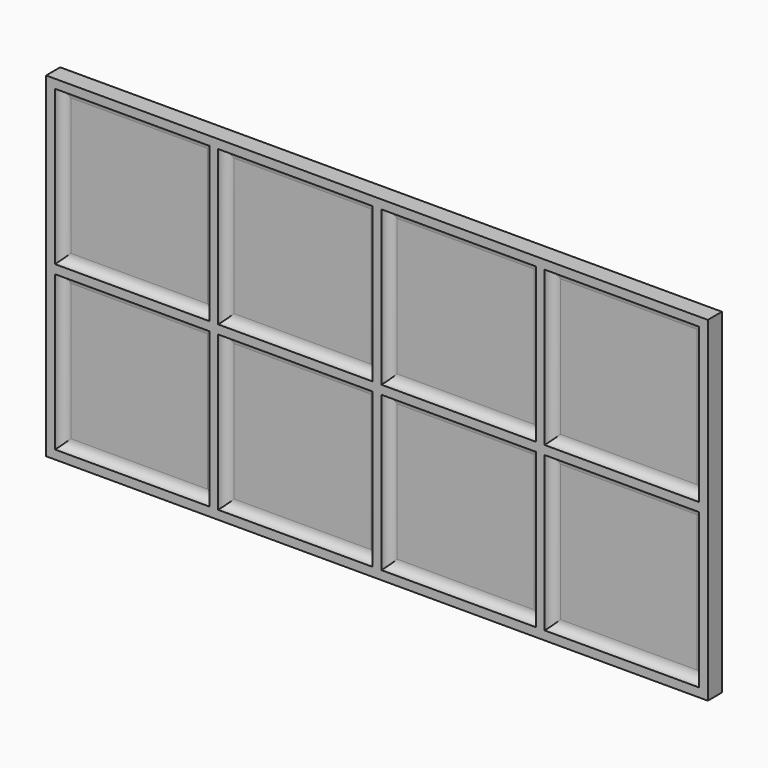
from build123d import *

# Parameters (mm, degrees)
F0_W     = 150
F0_H     = 76
F0_W_2   = 35
F0_H_2   = 35
F1_DEPTH = 2
F2_DEPTH = 4
F3_R     = 1.99999


# Not quite as in the source:
# - a fillet or chamfer is up to 0.001 mm smaller than in the source, because OpenCascade refuses the exact size


with BuildPart() as f1:
    # F0 (on Front) → F1 (new body)
    with BuildSketch(Plane.XZ):
        Rectangle(F0_W, F0_H)
        with Locations((-55.5, -18.5)):
            Rectangle(F0_W_2, F0_H_2, mode=Mode.SUBTRACT)
        with Locations((-18.5, -18.5)):
            Rectangle(F0_W_2, F0_H_2, mode=Mode.SUBTRACT)
        with Locations((18.5, -18.5)):
            Rectangle(F0_W_2, F0_H_2, mode=Mode.SUBTRACT)
        with Locations((55.5, -18.5)):
            Rectangle(F0_W_2, F0_H_2, mode=Mode.SUBTRACT)
        with Locations((-55.5, 18.5)):
            Rectangle(F0_W_2, F0_H_2, mode=Mode.SUBTRACT)
        with Locations((-18.5, 18.5)):
            Rectangle(F0_W_2, F0_H_2, mode=Mode.SUBTRACT)
        with Locations((18.5, 18.5)):
            Rectangle(F0_W_2, F0_H_2, mode=Mode.SUBTRACT)
        with Locations((55.5, 18.5)):
            Rectangle(F0_W_2, F0_H_2, mode=Mode.SUBTRACT)
        with Locations((-55.5, -18.5)):
            Rectangle(F0_W_2, F0_H_2)
        with Locations((-55.5, 18.5)):
            Rectangle(F0_W_2, F0_H_2)
        with Locations((-18.5, 18.5)):
            Rectangle(F0_W_2, F0_H_2)
        with Locations((18.5, 18.5)):
            Rectangle(F0_W_2, F0_H_2)
        with Locations((55.5, -18.5)):
            Rectangle(F0_W_2, F0_H_2)
        with Locations((55.5, 18.5)):
            Rectangle(F0_W_2, F0_H_2)
        with Locations((18.5, -18.5)):
            Rectangle(F0_W_2, F0_H_2)
        with Locations((-18.5, -18.5)):
            Rectangle(F0_W_2, F0_H_2)
    extrude(amount=F1_DEPTH)

    # F0 (on Front) → F2 (join)
    with BuildSketch(Plane.XZ):
        Rectangle(F0_W, F0_H)
        with Locations((-55.5, -18.5)):
            Rectangle(F0_W_2, F0_H_2, mode=Mode.SUBTRACT)
        with Locations((-18.5, -18.5)):
            Rectangle(F0_W_2, F0_H_2, mode=Mode.SUBTRACT)
        with Locations((18.5, -18.5)):
            Rectangle(F0_W_2, F0_H_2, mode=Mode.SUBTRACT)
        with Locations((55.5, -18.5)):
            Rectangle(F0_W_2, F0_H_2, mode=Mode.SUBTRACT)
        with Locations((-55.5, 18.5)):
            Rectangle(F0_W_2, F0_H_2, mode=Mode.SUBTRACT)
        with Locations((-18.5, 18.5)):
            Rectangle(F0_W_2, F0_H_2, mode=Mode.SUBTRACT)
        with Locations((18.5, 18.5)):
            Rectangle(F0_W_2, F0_H_2, mode=Mode.SUBTRACT)
        with Locations((55.5, 18.5)):
            Rectangle(F0_W_2, F0_H_2, mode=Mode.SUBTRACT)
    extrude(amount=F2_DEPTH)

    # F3 (radius 2 in the source; OpenCascade refuses exactly that, so slightly less here)
    f3_edges = [f1.edges().sort_by_distance(p)[0] for p in [
        (-73, -2, -18.5),
        (-55.5, -2, -1),
        (-55.5, -2, 36),
        (-36, -2, 18.5),
        (-18.5, -2, 36),
        (-73, -2, 18.5),
        (1, -2, 18.5),
        (18.5, -2, 36),
        (38, -2, 18.5),
        (55.5, -2, 36),
        (55.5, -2, -1),
        (38, -2, -18.5),
        (18.5, -2, -1),
        (1, -2, -18.5),
        (-18.5, -2, -1),
        (-36, -2, -18.5),
        (73, -2, -18.5),
        (55.5, -2, -36),
        (18.5, -2, -36),
        (-18.5, -2, -36),
        (-55.5, -2, -36),
        (-38, -2, -18.5),
        (-1, -2, -18.5),
        (36, -2, -18.5),
        (55.5, -2, 1),
        (73, -2, 18.5),
        (18.5, -2, 1),
        (36, -2, 18.5),
        (-18.5, -2, 1),
        (-1, -2, 18.5),
        (-55.5, -2, 1),
        (-38, -2, 18.5),
    ]]
    fillet(f3_edges, radius=F3_R)


solid = f1.part
